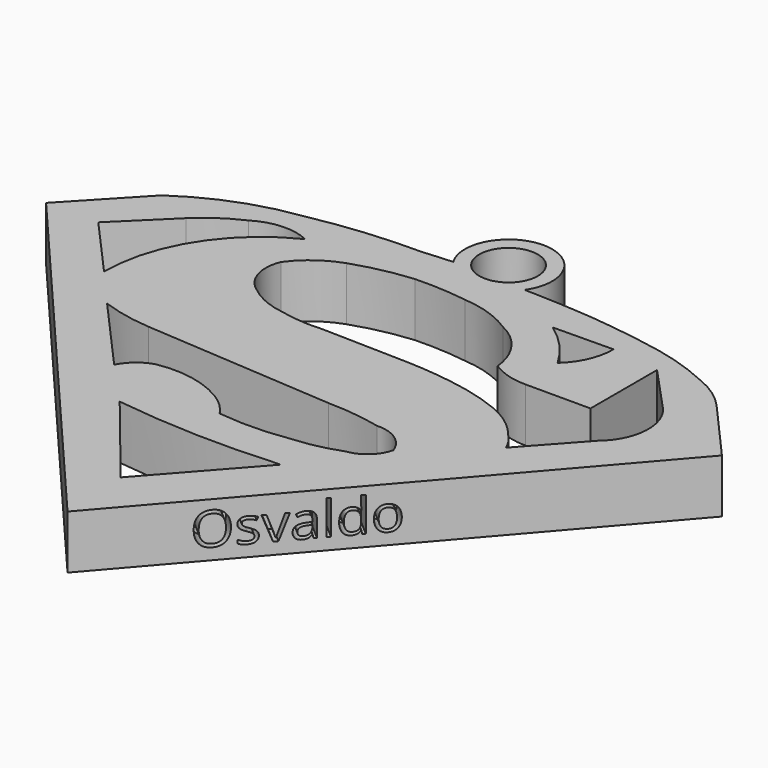
from build123d import *

# Parameters (mm, degrees)
F0_R         = 2.7211510446
F1_DEPTH     = 5
F2_TEXT_SIZE = 4.1932844195
F3_DEPTH     = 2


# Not quite as in the source:
# - Text() gives the source's letters only with a copy of the font that has no kerning and outlines rounded to 1/6400 em; it was checked with that copy


with BuildPart() as f1:
    # F0 (on Top) → F1 (new body)
    with BuildSketch(Plane.XY):
        with BuildLine():
            Line((7.1545867249, 43.9852103591), (1.3572657481, 37.8331281245))
            Line((1.3572657481, 37.8331281245), (32.8908823431, 0.9091482498))
            Line((32.8908823431, 0.9091482498), (64.4760280848, 37.4763384461))
            Line((64.4760280848, 37.4763384461), (59.3087077141, 43.3235689998))
            ThreePointArc((59.3087077141, 43.3235689998), (57.7475174136, 44.7202141939), (55.9045895934, 45.7159802318))
            ThreePointArc((55.9045895934, 45.7159802318), (53.3263457476, 46.7463657867), (50.6481789052, 47.4787987769))
            ThreePointArc((50.6481789052, 47.4787987769), (47.0553833366, 48.0961079899), (43.4366390109, 48.5364943743))
            ThreePointArc((43.4366390109, 48.5364943743), (41.0716120259, 48.6990790861), (38.7033598809, 48.8047588192))
            Line((38.7033598809, 48.8047588192), (37.0342921314, 48.8591432511))
            ThreePointArc((37.0342921314, 48.8591432511), (33.8132259951, 55.2077770871), (30.2312676623, 49.0555422785))
            Line((30.2312676623, 49.0555422785), (28.9305186751, 48.9716004974))
            ThreePointArc((28.9305186751, 48.9716004974), (28.2343518261, 48.9204722722), (27.5392010808, 48.8570071757))
            ThreePointArc((27.5392010808, 48.8570071757), (22.321550206, 48.6250976561), (17.1545874327, 47.8634163737))
            ThreePointArc((17.1545874327, 47.8634163737), (11.9242000649, 46.518369044), (7.1545867249, 43.9852103591))
        make_face()
        with BuildLine():
            Line((32.54615888, 7.514981553), (25.0456999691, 16.7770758271))
            ThreePointArc((25.0456999691, 16.7770758271), (32.7012103378, 16.166641098), (40.3789170086, 16.3463348368))
            Line((40.3789170086, 16.3463348368), (32.54615888, 7.514981553))
        make_face(mode=Mode.SUBTRACT)
        with BuildLine():
            ThreePointArc((29.8950225115, 21.7550303787), (26.7756800474, 22.974267053), (23.4265886247, 22.994812578))
            ThreePointArc((23.4265886247, 22.994812578), (22.069163024, 22.261642565), (21.1087334901, 21.0542827845))
            Line((21.1087334901, 21.0542827845), (14.6942026913, 28.2504167408))
            ThreePointArc((14.6942026913, 28.2504167408), (16.9647846824, 27.6047445169), (19.3029623479, 27.280151844))
            Line((19.3029623479, 27.280151844), (37.0103009045, 26.0673183948))
            ThreePointArc((37.0103009045, 26.0673183948), (39.5330778179, 25.9083041962), (42.0233383775, 25.4743788391))
            ThreePointArc((42.0233383775, 25.4743788391), (44.0562391064, 24.892043633), (45.3384108841, 23.2104267925))
            ThreePointArc((45.3384108841, 23.2104267925), (44.3892853906, 21.647665509), (42.7240841091, 20.8925716579))
            ThreePointArc((42.7240841091, 20.8925716579), (40.6691492303, 20.2801667377), (38.5465547442, 19.9762098491))
            ThreePointArc((38.5465547442, 19.9762098491), (35.2227339105, 19.6752710353), (31.8894572556, 19.8414511979))
            ThreePointArc((31.8894572556, 19.8414511979), (30.9980878089, 20.908561167), (29.8950225115, 21.7550303787))
        make_face(mode=Mode.SUBTRACT)
        with BuildLine():
            ThreePointArc((14.5681528375, 44.8600761592), (17.0538778934, 45.6356578866), (19.6081399918, 45.1295934618))
            ThreePointArc((19.6081399918, 45.1295934618), (13.6174192524, 39.760497185), (11.387838982, 32.0310145617))
            Line((11.387838982, 32.0310145617), (6.2250694058, 37.8144673821))
            Line((6.2250694058, 37.8144673821), (10.7948994264, 42.2996543348))
            ThreePointArc((10.7948994264, 42.2996543348), (12.5660907634, 43.7499805358), (14.5681528375, 44.8600761592))
        make_face(mode=Mode.SUBTRACT)
        with BuildLine():
            Line((52.4084940553, 37.2866168618), (52.4084940553, 45.0217872858))
            Line((52.4084940553, 45.0217872858), (56.6129758954, 40.4669307172))
            ThreePointArc((56.6129758954, 40.4669307172), (57.702640263, 36.9302908257), (55.9930838645, 33.6481258273))
            Line((55.9930838645, 33.6481258273), (51.4651797712, 28.6350883543))
            ThreePointArc((51.4651797712, 28.6350883543), (51.0078078723, 29.4980852331), (50.3871068358, 30.2521958947))
            ThreePointArc((50.3871068358, 30.2521958947), (48.7717515146, 31.8351157638), (46.8025170267, 32.9473763704))
            ThreePointArc((46.8025170267, 32.9473763704), (44.3488776793, 33.756462361), (41.816432029, 34.268014133))
            ThreePointArc((41.816432029, 34.268014133), (39.5718488904, 34.5427253162), (37.3141451032, 34.6707616775))
            Line((37.3141451032, 34.6707616775), (33.8886488316, 34.753276827))
            Line((33.8886488316, 34.753276827), (29.4186007231, 34.8609536886))
            ThreePointArc((29.4186007231, 34.8609536886), (27.3708917979, 34.8610028403), (25.3488775343, 35.1843759418))
            ThreePointArc((25.3488775343, 35.1843759418), (23.5247047427, 35.694553757), (21.8990445137, 36.6667248309))
            ThreePointArc((21.8990445137, 36.6667248309), (20.3722414873, 38.6893203958), (20.4706005752, 41.2215813994))
            ThreePointArc((20.4706005752, 41.2215813994), (22.1661015218, 42.9314760841), (24.2977570742, 44.0515242517))
            ThreePointArc((24.2977570742, 44.0515242517), (26.98420731, 44.7986090975), (29.7420211136, 45.2104508877))
            ThreePointArc((29.7420211136, 45.2104508877), (32.1872227524, 45.1854189136), (34.6202999353, 44.9409335852))
            ThreePointArc((34.6202999353, 44.9409335852), (37.1347972923, 44.4376035321), (39.4446738064, 43.3238223195))
            ThreePointArc((39.4446738064, 43.3238223195), (41.8736000104, 41.2686926188), (42.975358665, 38.2838360965))
            ThreePointArc((42.975358665, 38.2838360965), (44.5876022701, 37.5411555827), (46.3443361223, 37.2866168618))
            Line((46.3443361223, 37.2866168618), (52.4084940553, 37.2866168618))
        make_face(mode=Mode.SUBTRACT)
        with BuildLine():
            ThreePointArc((47.9075424373, 45.5877743661), (47.442394112, 43.2888505636), (46.0748188198, 41.383292526))
            ThreePointArc((46.0748188198, 41.383292526), (44.4231599912, 43.6576485052), (42.3195302532, 45.5218947151))
            Line((42.3195302532, 45.5218947151), (47.9075424373, 45.5877743661))
        make_face(mode=Mode.SUBTRACT)
        with Locations((33.696282655, 51.157001406)):
            Circle(F0_R, mode=Mode.SUBTRACT)
    extrude(amount=F1_DEPTH)

    # F2 (on face) → F3 (cut)
    with BuildSketch(Plane(origin=(18.3872952136, -15.8821445126, 0), x_dir=(0.6536719147, 0.7567780572, 0), z_dir=(0.7567780572, -0.6536719147, 0))):
        with Locations((31.2459971756, 1.09126186)):
            Text('Osvaldo', F2_TEXT_SIZE, font='Open Sans', text_align=(TextAlign.LEFT, TextAlign.BOTTOM))
    extrude(amount=-F3_DEPTH, mode=Mode.SUBTRACT)


solid = f1.part
